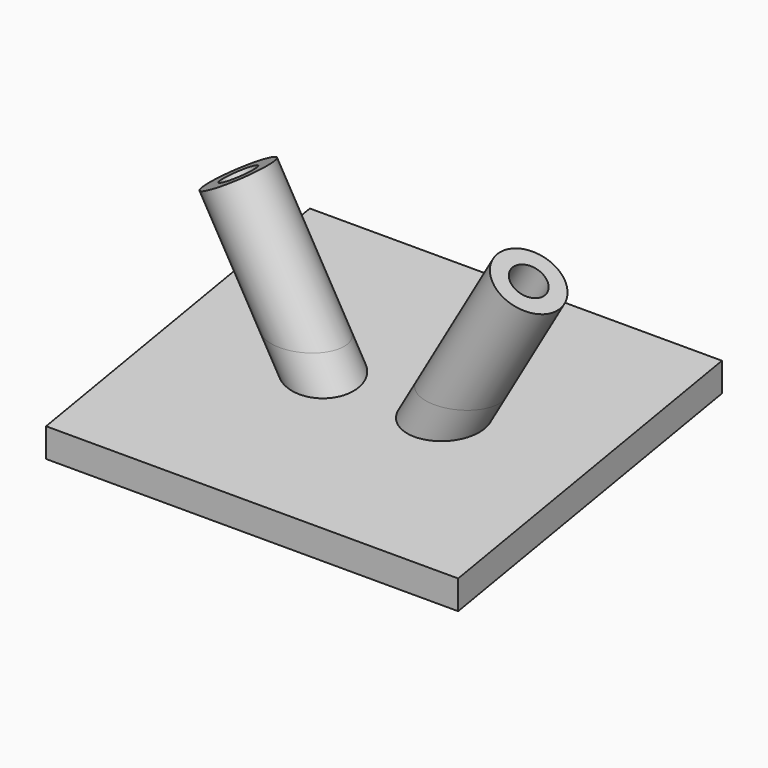
from build123d import *

# Parameters (mm, degrees)
F0_W         = 50
F0_H         = 40
F1_DEPTH     = 2.5
F7_R         = 4
F7_R_2       = 2.05
F10_DEPTH    = 8
F11_SIZE2    = 39.99999
F11_SIZE     = 6.99999
F6_R         = 2.05
F12_DEPTH    = 46.3
F13_R        = 2.05
F14_DEPTH    = 68.7
F15_T4_DEPTH = 50
F15_S5_R     = 4
F15_T6_DEPTH = 35
F15_S7_R     = 4
F15_T8_DEPTH = 35


# Not quite as in the source:
# - a fillet or chamfer that OpenCascade refuses, or shapes differently, is made with other operations: its cross-section is extruded or revolved along the edge and cut away or added
# - a fillet or chamfer is up to 0.001 mm smaller than in the source, because OpenCascade refuses the exact size


with BuildPart() as f1:
    # F0 (on Top) → F1 (new body)
    with BuildSketch(Plane.XY):
        Rectangle(F0_W, F0_H)
    extrude(amount=F1_DEPTH)

    # F7 (on offset) → F8 (join, up to the last surface of F1)
    with BuildSketch(Plane(origin=(-11.6521931986, 0, 20.1821906397), x_dir=(0.8660254038, 0, 0.5), z_dir=(0.5, 0, -0.8660254038))):
        with Locations((-6.8889131071, 0.075317279)):
            Circle(F7_R)
        with Locations((-6.8889131071, 0.075317279)):
            Circle(F7_R_2, mode=Mode.SUBTRACT)
    extrude(until=Until.LAST)

    # F9: F1 across plane


with BuildPart() as f1_1:
    add(f1.part)
    add(f1.part.mirror(Plane.YZ))

    # F0 (on Top) → F10 (join)
    with BuildSketch(Plane.XY):
        Rectangle(F0_W, F0_H)
    extrude(amount=-F10_DEPTH)

    # F11 (size 7 and 40 in the source; OpenCascade refuses exactly that, so slightly less here)
    f11_edges = [f1_1.edges().sort_by_distance(p)[0] for p in [
        (0, 20, -8),
    ]]
    f11_side = f1_1.faces().sort_by_distance((0, 20, -2.75))[0]
    chamfer(f11_edges, length=F11_SIZE, length2=F11_SIZE2, reference=f11_side)

    # F6 (on offset) → F12 (cut)
    with BuildSketch(Plane(origin=(-11.6521931986, 0, 20.1821906397), x_dir=(0.8660254038, 0, 0.5), z_dir=(0.5, 0, -0.8660254038))):
        with Locations((-6.8571413867, 0.094557312)):
            Circle(F6_R)
    extrude(amount=F12_DEPTH, mode=Mode.SUBTRACT)

    # F13 (on offset) → F14 (cut)
    with BuildSketch(Plane(origin=(11.6521931986, 0, 20.1821906397), x_dir=(0.8660254038, 0, -0.5), z_dir=(0.5, 0, 0.8660254038))):
        with Locations((6.8889131072, -0.075317279)):
            Circle(F13_R)
    extrude(amount=-F14_DEPTH, mode=Mode.SUBTRACT)

    # F15: chamfer of 7 x 40 on 1 edges, made by hand


with BuildPart() as f15_tool2:
    # F15_s3 → F15_t4 (new body)
    with BuildSketch(Plane.YZ.offset(-25)):
        with BuildLine():
            Line((21.5760487474, 2.7758085308), (-21.5760487474, -4.7758085308))
            Line((-21.5760487474, -4.7758085308), (-22.3760487474, -4.7758085308))
            ThreePointArc((-22.3760487474, -4.7758085308), (-20.8, -1.1379042654), (-20.8, 2.5))
            Line((-20.8, 2.5), (-20, 3.3))
            ThreePointArc((-20, 3.3), (0.7880243737, 3.3), (21.5760487474, 3.5758085308))
            Line((21.5760487474, 3.5758085308), (21.5760487474, 2.7758085308))
        make_face()
    extrude(amount=F15_T4_DEPTH)

    # F15_s5 → F15_t6 (cut, symmetric)
    with BuildSketch(Plane(origin=(0.25, 0, -0.4330127019), x_dir=(0, 1, 0), z_dir=(-0.5, 0, 0.8660254038))):
        with Locations((-0.075317279, 6.8889131071)):
            Circle(F15_S5_R)
    extrude(amount=F15_T6_DEPTH, both=True, mode=Mode.SUBTRACT)

    # F15_s7 → F15_t8 (cut, symmetric)
    with BuildSketch(Plane(origin=(-0.25, 0, -0.4330127019), x_dir=(0, 1, 0), z_dir=(0.5, 0, 0.8660254038))):
        with Locations((-0.075317279, -6.8889131071)):
            Circle(F15_S7_R)
    extrude(amount=F15_T8_DEPTH, both=True, mode=Mode.SUBTRACT)


with BuildPart() as f1_2:
    add(f1_1.part)

    # F15_t1: cut F15_tool2
    add(f15_tool2.part, mode=Mode.SUBTRACT)


solid = f1_2.part
